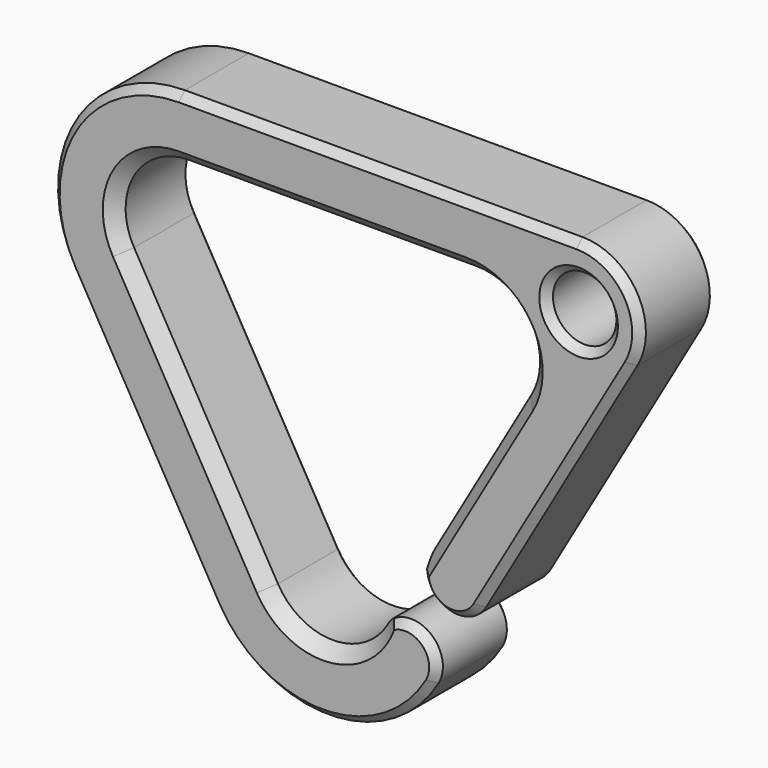
from build123d import *

# Parameters (mm, degrees)
F1_DEPTH     = 9.525
F3_T1_DEPTH  = 28.8029547439
F3_T3_DEPTH  = 22.5439921386
F3_T5_DEPTH  = 28.8029547439
F3_T8_ANGLE  = 120
F3_T10_ANGLE = 120
F3_T12_ANGLE = 149.490366343
F5_DEPTH     = 9.525
F6_SIZE      = 0.762
F8_R         = 3.175
F9_DEPTH     = 9.526
F10_SIZE     = 0.762
F12_DEPTH    = 1.27


# Not quite as in the source:
# - a fillet or chamfer that OpenCascade refuses, or shapes differently, is made with other operations: its cross-section is extruded or revolved along the edge and cut away or added
# - a feature of the source that left no trace in its solid (it failed there, or was rolled back) is left out
# - a feature names something its author has since deleted; it is built from what else it names


with BuildPart() as f1:
    # F0 (on Front) → F1 (new body)
    with BuildSketch(Plane.XZ):
        with BuildLine():
            Line((-14.4014773719, 43.9940905122), (14.4014773719, 43.9940905122))
            ThreePointArc((14.4014773719, 43.9940905122), (19.900738686, 40.8190905122), (19.900738686, 34.4690905122))
            Line((19.900738686, 34.4690905122), (10.261761314, 17.773891971))
            ThreePointArc((10.261761314, 17.773891971), (11.423891971, 13.436761314), (15.7610226281, 14.598891971))
            Line((15.7610226281, 14.598891971), (25.4, 31.2940905122))
            ThreePointArc((25.4, 31.2940905122), (25.4, 43.9940905122), (14.4014773719, 50.3440905122))
            Line((14.4014773719, 50.3440905122), (-14.4014773719, 50.3440905122))
            ThreePointArc((-14.4014773719, 50.3440905122), (-25.4, 43.9940905122), (-25.4, 31.2940905122))
            Line((-25.4, 31.2940905122), (-10.9985226281, 6.35))
            ThreePointArc((-10.9985226281, 6.35), (0, 0), (10.9985226281, 6.35))
            ThreePointArc((10.9985226281, 6.35), (9.836391971, 10.687130657), (5.499261314, 9.525))
            ThreePointArc((5.499261314, 9.525), (0, 6.35), (-5.499261314, 9.525))
            Line((-5.499261314, 9.525), (-19.900738686, 34.4690905122))
            ThreePointArc((-19.900738686, 34.4690905122), (-19.900738686, 40.8190905122), (-14.4014773719, 43.9940905122))
        make_face()
    extrude(amount=F1_DEPTH)

    # F3: chamfer of 1.27 on 6 edges, made by hand

    # F3_s2 → F3_t1 (cut)
    with BuildSketch(Plane.YZ.offset(-14.4014773719)):
        Polygon((-8.255, 43.9940905122), (-9.525, 45.2640905122), (-9.525, 43.9940905122), align=None)
    extrude(amount=F3_T1_DEPTH, mode=Mode.SUBTRACT)

    # F3_s4 → F3_t3 (cut)
    with BuildSketch(Plane(origin=(19.900738686, 0, 34.4690905122), x_dir=(0, 1, 0), z_dir=(-0.5, 0, -0.8660254038))):
        Polygon((-8.255, 0), (-9.525, 1.27), (-9.525, 0), align=None)
    extrude(amount=F3_T3_DEPTH, mode=Mode.SUBTRACT)

    # F3_s6 → F3_t5 (cut)
    with BuildSketch(Plane(origin=(-5.499261314, 0, 9.525), x_dir=(0, 1, 0), z_dir=(-0.5, 0, 0.8660254038))):
        Polygon((-8.255, 0), (-9.525, 1.27), (-9.525, 0), align=None)
    extrude(amount=F3_T5_DEPTH, mode=Mode.SUBTRACT)

    # F3_s7 → F3_t8 (revolve, cut)
    with BuildSketch(Plane(origin=(-19.900738686, 0, 34.4690905122), x_dir=(0, 1, 0), z_dir=(0.5, 0, -0.8660254038))):
        Polygon((-8.255, 0), (-9.525, -1.27), (-9.525, 0), align=None)
    revolve(axis=Axis((-14.4014773719, -9.525, 37.6440905122), (0, 1, 0)), revolution_arc=F3_T8_ANGLE, mode=Mode.SUBTRACT)

    # F3_s9 → F3_t10 (revolve, cut)
    with BuildSketch(Plane.YZ.offset(14.4014773719)):
        Polygon((-8.255, 43.9940905122), (-9.525, 45.2640905122), (-9.525, 43.9940905122), align=None)
    revolve(axis=Axis((14.4014773719, -9.525, 37.6440905122), (0, 1, 0)), revolution_arc=F3_T10_ANGLE, mode=Mode.SUBTRACT)

    # F3_s11 → F3_t12 (revolve, cut)
    with BuildSketch(Plane(origin=(0.1129578151, 0, 12.698995238), x_dir=(0, 1, 0), z_dir=(0.008894668, 0, 0.9999604417))):
        Polygon((-8.255, -6.2370377163), (-9.525, -7.5070377163), (-9.525, -6.2370377163), align=None)
    revolve(axis=Axis((0, -9.525, 12.7), (0, 1, 0)), revolution_arc=F3_T12_ANGLE, mode=Mode.SUBTRACT)

    # F4 (on face) → F5 (join, through all)
    with BuildSketch(Plane(origin=(0, 0, 0), x_dir=(-1, 0, 0), z_dir=(0, 1, 0))):
        with BuildLine():
            Line((-30.899261314, 40.8190905122), (-25.4, 31.2940905122))
            ThreePointArc((-25.4, 31.2940905122), (-25.4, 43.9940905122), (-14.4014773719, 50.3440905122))
            Line((-14.4014773719, 50.3440905122), (-25.4, 50.3440905122))
            ThreePointArc((-25.4, 50.3440905122), (-30.899261314, 47.1690905122), (-30.899261314, 40.8190905122))
        make_face()
    extrude(amount=-F5_DEPTH)

    # F6
    f6_edges = [f1.edges().sort_by_distance(p)[0] for p in [
        (12.821161, -9.525, 13.017096),
        (23.330142, -9.525, 27.708991),
        (30.899261, -9.525, 47.169091),
        (5.499261, -9.525, 50.344091),
        (-25.4, -9.525, 43.994091),
        (-18.199261, -9.525, 18.822045),
        (0, -9.525, 0),
        (10.76839, -9.525, 9.869534),
        (9.836392, 0, 10.687131),
        (0, 0, 0),
        (-18.199261, 0, 18.822045),
        (-25.4, 0, 43.994091),
        (5.499261, 0, 50.344091),
        (30.899261, 0, 47.169091),
        (23.330142, 0, 27.708991),
        (11.423892, 0, 13.436761),
        (15.08125, 0, 26.121491),
        (19.900739, 0, 40.819091),
        (0, 0, 43.994091),
        (-19.900739, 0, 40.819091),
        (-12.7, 0, 21.997045),
        (0, 0, 6.35),
    ]]
    chamfer(f6_edges, length=F6_SIZE)

    # F8 (on face) → F9 (cut, through all)
    with BuildSketch(Plane.XZ.offset(9.525)):
        with Locations((25.6199704526, 44.1210905122)):
            Circle(F8_R)
    extrude(amount=-F9_DEPTH, mode=Mode.SUBTRACT)

    # F10
    f10_edges = [f1.edges().sort_by_distance(p)[0] for p in [
        (22.44497, -9.525, 44.121091),
        (28.79497, -4.7625, 44.121091),
        (22.44497, 0, 44.121091),
    ]]
    chamfer(f10_edges, length=F10_SIZE)

    # F11 (on offset) → F12 (join)
    with BuildSketch(Plane(origin=(0, -0.762, 0), x_dir=(-1, 0, 0), z_dir=(0, 1, 0))):
        with BuildLine():
            Line((-19.900738686, 34.4690905122), (-14.4014773719, 43.9940905122))
            ThreePointArc((-14.4014773719, 43.9940905122), (-19.900738686, 40.8190905122), (-19.900738686, 34.4690905122))
        make_face()
    extrude(amount=-F12_DEPTH)


solid = f1.part
